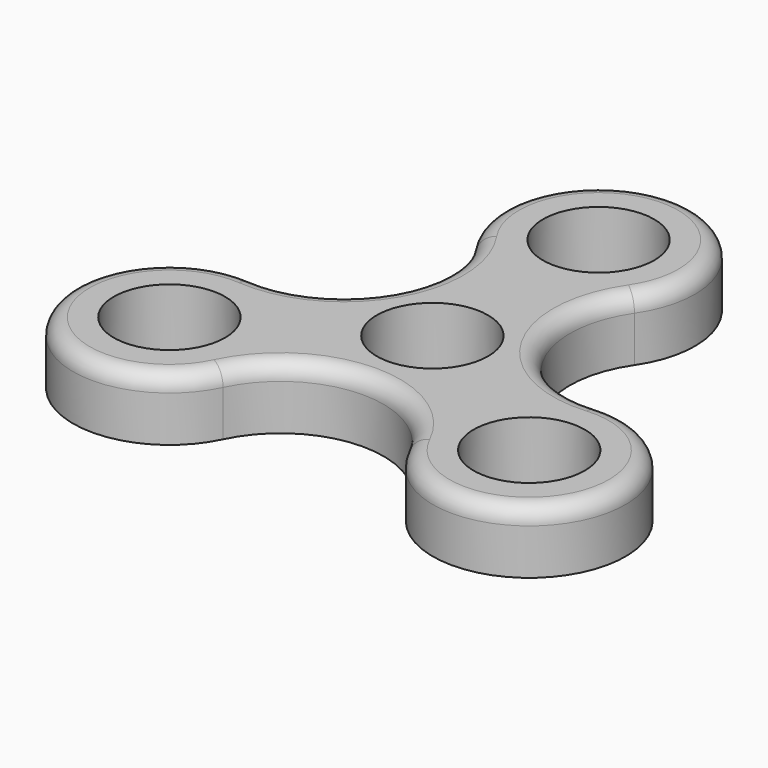
from build123d import *

# Parameters (mm, degrees)
F0_R     = 8.5
F1_DEPTH = 9.525
F2_R     = 2.54


# Not quite as in the source:
# - a feature names something its author has since deleted; it is built from what else it names


with BuildPart() as f1:
    # F0 (on Top) → F1 (new body)
    with BuildSketch(Plane.XY):
        with BuildLine():
            ThreePointArc((-12.1502250441, 23.4191023666), (-11.5002285841, 6.6396600688), (-26.3566501053, -1.1871476334))
            ThreePointArc((-26.3566501053, -1.1871476334), (-40.2545928187, -23.241), (-14.2064250612, -22.2319547331))
            ThreePointArc((-14.2064250612, -22.2319547331), (0, -13.2793201375), (14.2064250612, -22.2319547331))
            ThreePointArc((14.2064250612, -22.2319547331), (40.2545928187, -23.241), (26.3566501053, -1.1871476334))
            ThreePointArc((26.3566501053, -1.1871476334), (11.5002285841, 6.6396600688), (12.1502250441, 23.4191023666))
            ThreePointArc((12.1502250441, 23.4191023666), (0, 46.482), (-12.1502250441, 23.4191023666))
        make_face()
        with Locations((-27.4963065702, -15.875)):
            Circle(F0_R, mode=Mode.SUBTRACT)
        with Locations((27.4963065702, -15.875)):
            Circle(F0_R, mode=Mode.SUBTRACT)
        Circle(F0_R, mode=Mode.SUBTRACT)
        with Locations((0, 31.75)):
            Circle(F0_R, mode=Mode.SUBTRACT)
    extrude(amount=F1_DEPTH)

    # F2
    f2_edges = [f1.edges().sort_by_distance(p)[0] for p in [
        (-11.500229, 6.63966, 9.525),
    ]]
    fillet(f2_edges, radius=F2_R)


solid = f1.part
